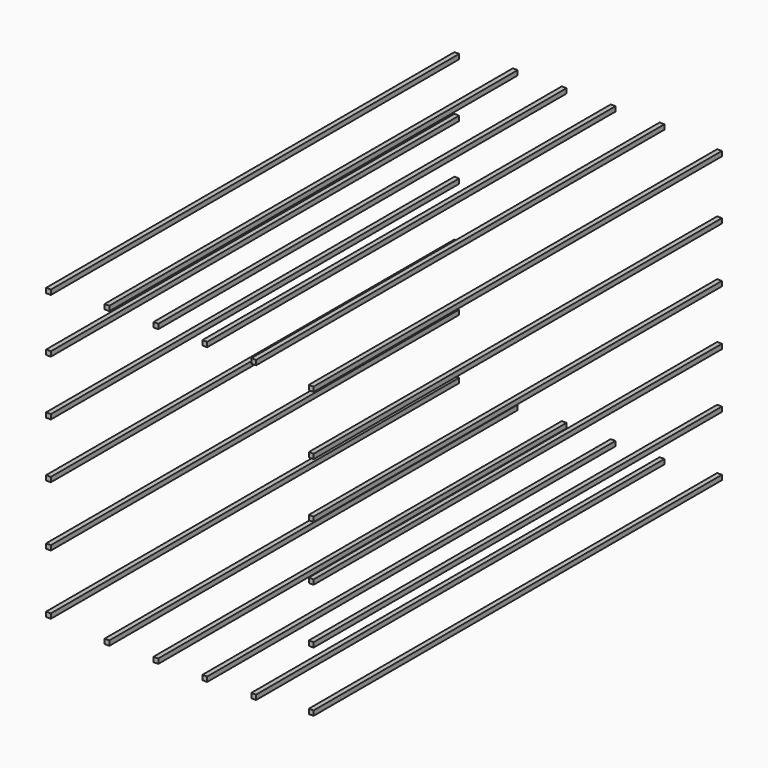
from build123d import *

# Parameters (mm, degrees)
F0_W     = 45
F0_H     = 45
F2_DEPTH = 4800


# Not quite as in the source:
# - a feature of the source that left no trace in its solid (it failed there, or was rolled back) is left out


with BuildPart() as f2:
    # F0 (on Front) → F2 (new body)
    with BuildSketch(Plane.XZ):
        with Locations((-35.5, 2690.5)):
            Rectangle(F0_W, F0_H)
    extrude(amount=F2_DEPTH)


with BuildPart() as f2b:
    # F0 (on Front) → F2, piece 2 (new body)
    with BuildSketch(Plane.XZ):
        with Locations((2435.5, 2690.5)):
            Rectangle(F0_W, F0_H)
    extrude(amount=F2_DEPTH)


with BuildPart() as f2c:
    # F0 (on Front) → F2, piece 3 (new body)
    with BuildSketch(Plane.XZ):
        with Locations((514.5, 2735.5)):
            Rectangle(F0_W, F0_H)
    extrude(amount=F2_DEPTH)


with BuildPart() as f2d:
    # F0 (on Front) → F2, piece 4 (new body)
    with BuildSketch(Plane.XZ):
        with Locations((974.5, 2735.5)):
            Rectangle(F0_W, F0_H)
    extrude(amount=F2_DEPTH)


with BuildPart() as f2e:
    # F0 (on Front) → F2, piece 5 (new body)
    with BuildSketch(Plane.XZ):
        with Locations((1434.5, 2735.5)):
            Rectangle(F0_W, F0_H)
    extrude(amount=F2_DEPTH)


with BuildPart() as f2f:
    # F0 (on Front) → F2, piece 6 (new body)
    with BuildSketch(Plane.XZ):
        with Locations((1894.5, 2735.5)):
            Rectangle(F0_W, F0_H)
    extrude(amount=F2_DEPTH)


with BuildPart() as f2g:
    # F0 (on Front) → F2, piece 7 (new body)
    with BuildSketch(Plane.XZ):
        with Locations((-35.5, 2179.5)):
            Rectangle(F0_W, F0_H)
    extrude(amount=F2_DEPTH)


with BuildPart() as f2h:
    # F0 (on Front) → F2, piece 8 (new body)
    with BuildSketch(Plane.XZ):
        with Locations((-35.5, 1659.5)):
            Rectangle(F0_W, F0_H)
    extrude(amount=F2_DEPTH)


with BuildPart() as f2i:
    # F0 (on Front) → F2, piece 9 (new body)
    with BuildSketch(Plane.XZ):
        with Locations((-35.5, 1139.5)):
            Rectangle(F0_W, F0_H)
    extrude(amount=F2_DEPTH)


with BuildPart() as f2j:
    # F0 (on Front) → F2, piece 10 (new body)
    with BuildSketch(Plane.XZ):
        with Locations((-35.5, 574.5)):
            Rectangle(F0_W, F0_H)
    extrude(amount=F2_DEPTH)


with BuildPart() as f2k:
    # F0 (on Front) → F2, piece 11 (new body)
    with BuildSketch(Plane.XZ):
        with Locations((-35.5, 9.5)):
            Rectangle(F0_W, F0_H)
    extrude(amount=F2_DEPTH)


with BuildPart() as f2l:
    # F0 (on Front) → F2, piece 12 (new body)
    with BuildSketch(Plane.XZ):
        with Locations((2435.5, 9.5)):
            Rectangle(F0_W, F0_H)
    extrude(amount=F2_DEPTH)


with BuildPart() as f2m:
    # F0 (on Front) → F2, piece 13 (new body)
    with BuildSketch(Plane.XZ):
        with Locations((2435.5, 574.5)):
            Rectangle(F0_W, F0_H)
    extrude(amount=F2_DEPTH)


with BuildPart() as f2n:
    # F0 (on Front) → F2, piece 14 (new body)
    with BuildSketch(Plane.XZ):
        with Locations((2435.5, 1094.5)):
            Rectangle(F0_W, F0_H)
    extrude(amount=F2_DEPTH)


with BuildPart() as f2o:
    # F0 (on Front) → F2, piece 15 (new body)
    with BuildSketch(Plane.XZ):
        with Locations((2435.5, 1614.5)):
            Rectangle(F0_W, F0_H)
    extrude(amount=F2_DEPTH)


with BuildPart() as f2p:
    # F0 (on Front) → F2, piece 16 (new body)
    with BuildSketch(Plane.XZ):
        with Locations((2435.5, 2134.5)):
            Rectangle(F0_W, F0_H)
    extrude(amount=F2_DEPTH)


with BuildPart() as f2q:
    # F0 (on Front) → F2, piece 17 (new body)
    with BuildSketch(Plane.XZ):
        with Locations((514.5, -35.5)):
            Rectangle(F0_W, F0_H)
    extrude(amount=F2_DEPTH)


with BuildPart() as f2r:
    # F0 (on Front) → F2, piece 18 (new body)
    with BuildSketch(Plane.XZ):
        with Locations((974.5, -35.5)):
            Rectangle(F0_W, F0_H)
    extrude(amount=F2_DEPTH)


with BuildPart() as f2s:
    # F0 (on Front) → F2, piece 19 (new body)
    with BuildSketch(Plane.XZ):
        with Locations((1434.5, -35.5)):
            Rectangle(F0_W, F0_H)
    extrude(amount=F2_DEPTH)


with BuildPart() as f2t:
    # F0 (on Front) → F2, piece 20 (new body)
    with BuildSketch(Plane.XZ):
        with Locations((1894.5, -35.5)):
            Rectangle(F0_W, F0_H)
    extrude(amount=F2_DEPTH)


solid = Compound([f2.part, f2b.part, f2c.part, f2d.part, f2e.part, f2f.part, f2g.part, f2h.part, f2i.part, f2j.part, f2k.part, f2l.part, f2m.part, f2n.part, f2o.part, f2p.part, f2q.part, f2r.part, f2s.part, f2t.part])
